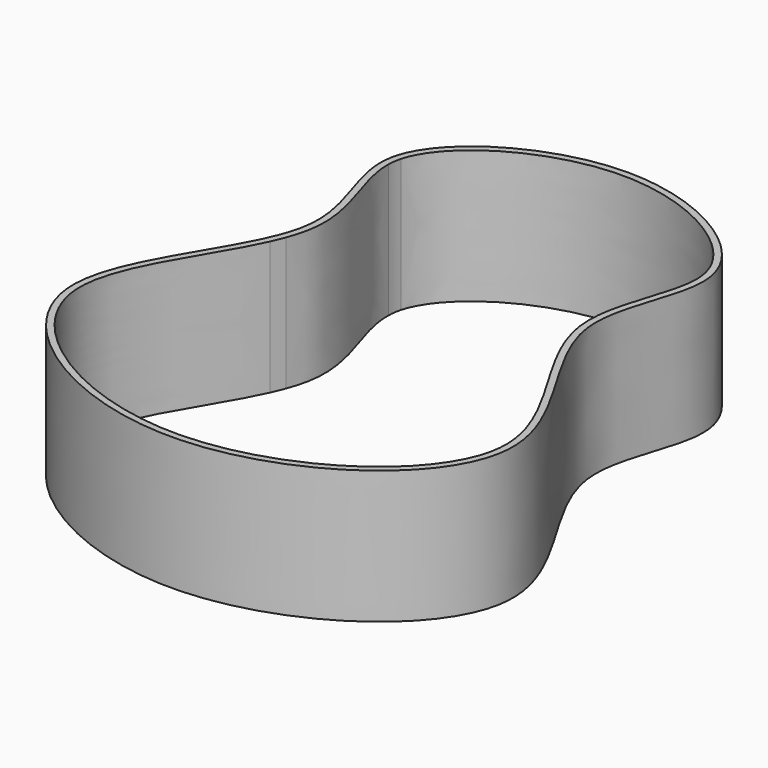
from build123d import *

# Parameters (mm, degrees)
F5_DEPTH = 63.5


# Not quite as in the source:
# - the dataset's text gives a spline's control points without its knots; the knots are read off the source's solid


with BuildPart() as f5:
    # F2 (on Top) → F5 (new body, through all)
    with BuildSketch(Plane.XY):
        with BuildLine():
            add(Edge.make_bspline(
                [(0, 107.95), (-35.4120909188, 107.95), (-101.0360842003, 68.1188915444), (-41.6735084728, -2.8361549385), (-147.9467406323, -100.2012664435), (0, -199.2106394656), (147.9467406323, -100.2012664435), (41.6735084728, -2.8361549385), (101.0360842003, 68.1188915444), (35.4120909188, 107.95), (0, 107.95)],
                knots=[0, 0, 0, 0, 0.1211744653, 0.2245547239, 0.3552265354, 0.5, 0.6447734646, 0.7754452761, 0.8788255347, 1, 1, 1, 1], degree=3))
        make_face()
        with BuildLine():
            add(Edge.make_bspline(
                [(0, 104.775), (-2.2017481327, 104.775), (-6.6052443982, 104.6027636289), (-15.371540612, 103.6082428137), (-26.1163430628, 101.2207379951), (-38.2681973915, 96.7746422098), (-49.2709251868, 91.0117607618), (-57.1445580694, 85.3455999483), (-62.4673341969, 80.4474462476), (-65.9238639338, 76.6330861755), (-68.8001393736, 72.7213984058), (-71.0564914793, 68.7584001979), (-72.3017219402, 65.6767963474), (-72.8136631637, 63.9301750524), (-72.9278134841, 63.5000063505)],
                knots=[0, 0, 0, 0, 0.0078125, 0.015625, 0.03125, 0.046875, 0.0625, 0.078125, 0.0859375, 0.09375, 0.1015625, 0.109375, 0.1171875, 0.119741505, 0.119741505, 0.119741505, 0.119741505], degree=3))
            add(Edge.make_bspline(
                [(72.9278134841, 63.5000063505), (72.8136631637, 63.9301750524), (72.3017219402, 65.6767963474), (71.0564914793, 68.7584001979), (68.8001393736, 72.7213984058), (65.9238639338, 76.6330861755), (62.4673341969, 80.4474462476), (57.1445580694, 85.3455999483), (49.2709251868, 91.0117607618), (38.2681973915, 96.7746422098), (26.1163430628, 101.2207379951), (15.371540612, 103.6082428137), (6.6052443982, 104.6027636289), (2.2017481327, 104.775), (0, 104.775)],
                knots=[0.880258495, 0.880258495, 0.880258495, 0.880258495, 0.8828125, 0.890625, 0.8984375, 0.90625, 0.9140625, 0.921875, 0.9375, 0.953125, 0.96875, 0.984375, 0.9921875, 1, 1, 1, 1], degree=3))
            add(Edge.make_bspline(
                [(73.7979876463, 57.1499999799), (73.7718089647, 58.3956160725), (73.6148935537, 60.2937642863), (73.2102216519, 62.3867267954), (72.9882515794, 63.2722489783), (72.9278134841, 63.5000063505)],
                knots=[0.8678367594, 0.8678367594, 0.8678367594, 0.8678367594, 0.875, 0.87890625, 0.880258495, 0.880258495, 0.880258495, 0.880258495], degree=3))
            add(Edge.make_bspline(
                [(66.7291899942, -12.7000033495), (66.0958270146, -10.9875159701), (65.217269308, -8.3297436688), (64.290069722, -4.7256477635), (63.7216918103, -1.8876036945), (63.3325778212, 0.9537204509), (63.1281778007, 3.7615979172), (63.0893891666, 6.5362776041), (63.2384551748, 10.1882294857), (63.7603381489, 14.6614399223), (64.7958827235, 19.8816564814), (66.5579017078, 26.6525019309), (69.1773452318, 34.7799177225), (71.5965196213, 42.4890054809), (72.9893709157, 48.3932067915), (73.6673321547, 52.6830830541), (73.8232156043, 55.563833003), (73.8003604207, 57.0371002541), (73.7979876463, 57.1499999799)],
                knots=[0.7585577924, 0.7585577924, 0.7585577924, 0.7585577924, 0.765625, 0.76953125, 0.7734375, 0.77734375, 0.78125, 0.78515625, 0.7890625, 0.796875, 0.8046875, 0.8125, 0.828125, 0.84375, 0.8515625, 0.859375, 0.8671875, 0.8678367594, 0.8678367594, 0.8678367594, 0.8678367594], degree=3))
            add(Edge.make_bspline(
                [(69.3614532719, -19.0500001132), (69.3426167016, -19.0086385189), (68.4615054488, -17.0707981023), (67.5715581082, -14.954379658), (66.7959830788, -12.8805985502), (66.7291899942, -12.7000033495)],
                knots=[0.749829616, 0.749829616, 0.749829616, 0.749829616, 0.75, 0.7578125, 0.7585577924, 0.7585577924, 0.7585577924, 0.7585577924], degree=3))
            add(Edge.make_bspline(
                [(-69.3614532719, -19.0500001132), (-70.2063170173, -20.9051632784), (-72.0386726478, -24.6608400473), (-76.1047789171, -32.2335128923), (-81.7086762924, -41.7903671927), (-88.4859214528, -53.2902266792), (-94.5830259686, -64.7550195426), (-98.4936842191, -74.1960733248), (-100.5801378169, -81.6181080241), (-101.5478394514, -87.1046098292), (-101.7973544457, -91.6066056278), (-101.628757954, -95.1651641691), (-101.2018148356, -98.7159700534), (-100.1923411379, -103.1573595965), (-98.2480737504, -108.4628346187), (-95.6008842173, -113.7151687278), (-91.179821607, -120.5995838786), (-84.0759861131, -128.8891422039), (-73.366446899, -138.033559619), (-60.8364043051, -146.0931924242), (-46.8583381525, -152.8014594446), (-31.8075746749, -157.9031399264), (-18.6854818735, -160.6106654852), (-8.0257679073, -161.731838197), (0, -162.0215809015), (8.0257679073, -161.731838197), (18.6854818735, -160.6106654852), (31.8075746749, -157.9031399264), (46.8583381525, -152.8014594446), (60.8364043051, -146.0931924242), (73.366446899, -138.033559619), (84.0759861131, -128.8891422039), (91.179821607, -120.5995838786), (95.6008842173, -113.7151687278), (98.2480737504, -108.4628346187), (100.1923411379, -103.1573595965), (101.2018148356, -98.7159700534), (101.628757954, -95.1651641691), (101.7973544457, -91.6066056278), (101.5478394514, -87.1046098292), (100.5801378169, -81.6181080241), (98.4936842191, -74.1960733248), (94.5830259686, -64.7550195426), (88.4859214528, -53.2902266792), (81.7086762924, -41.7903671927), (76.1047789171, -32.2335128923), (72.0386726478, -24.6608400473), (70.2063170173, -20.9051632784), (69.3614532719, -19.0500001132)],
                knots=[0.250170384, 0.250170384, 0.250170384, 0.250170384, 0.2578125, 0.265625, 0.28125, 0.296875, 0.3125, 0.328125, 0.3359375, 0.34375, 0.3515625, 0.35546875, 0.359375, 0.3671875, 0.375, 0.3828125, 0.390625, 0.40625, 0.421875, 0.4375, 0.453125, 0.46875, 0.484375, 0.4921875, 0.5, 0.5078125, 0.515625, 0.53125, 0.546875, 0.5625, 0.578125, 0.59375, 0.609375, 0.6171875, 0.625, 0.6328125, 0.640625, 0.64453125, 0.6484375, 0.65625, 0.6640625, 0.671875, 0.6875, 0.703125, 0.71875, 0.734375, 0.7421875, 0.749829616, 0.749829616, 0.749829616, 0.749829616], degree=3))
            add(Edge.make_bspline(
                [(-66.7291899942, -12.7000033495), (-66.7959830788, -12.8805985502), (-67.5715581082, -14.954379658), (-68.4615054488, -17.0707981023), (-69.3426167016, -19.0086385189), (-69.3614532719, -19.0500001132)],
                knots=[0.2414422076, 0.2414422076, 0.2414422076, 0.2414422076, 0.2421875, 0.25, 0.250170384, 0.250170384, 0.250170384, 0.250170384], degree=3))
            add(Edge.make_bspline(
                [(-73.7979876463, 57.1499999799), (-73.8003604207, 57.0371002541), (-73.8232156043, 55.563833003), (-73.6673321547, 52.6830830541), (-72.9893709157, 48.3932067915), (-71.5965196213, 42.4890054809), (-69.1773452318, 34.7799177225), (-66.5579017078, 26.6525019309), (-64.7958827235, 19.8816564814), (-63.7603381489, 14.6614399223), (-63.2384551748, 10.1882294857), (-63.0893891666, 6.5362776041), (-63.1281778007, 3.7615979172), (-63.3325778212, 0.9537204509), (-63.7216918103, -1.8876036945), (-64.290069722, -4.7256477635), (-65.217269308, -8.3297436688), (-66.0958270146, -10.9875159701), (-66.7291899942, -12.7000033495)],
                knots=[0.1321632406, 0.1321632406, 0.1321632406, 0.1321632406, 0.1328125, 0.140625, 0.1484375, 0.15625, 0.171875, 0.1875, 0.1953125, 0.203125, 0.2109375, 0.21484375, 0.21875, 0.22265625, 0.2265625, 0.23046875, 0.234375, 0.2414422076, 0.2414422076, 0.2414422076, 0.2414422076], degree=3))
            add(Edge.make_bspline(
                [(-72.9278134841, 63.5000063505), (-72.9882515794, 63.2722489783), (-73.2102216519, 62.3867267954), (-73.6148935537, 60.2937642863), (-73.7718089647, 58.3956160725), (-73.7979876463, 57.1499999799)],
                knots=[0.119741505, 0.119741505, 0.119741505, 0.119741505, 0.12109375, 0.125, 0.1321632406, 0.1321632406, 0.1321632406, 0.1321632406], degree=3))
        make_face(mode=Mode.SUBTRACT)
    extrude(amount=-F5_DEPTH)


solid = f5.part
